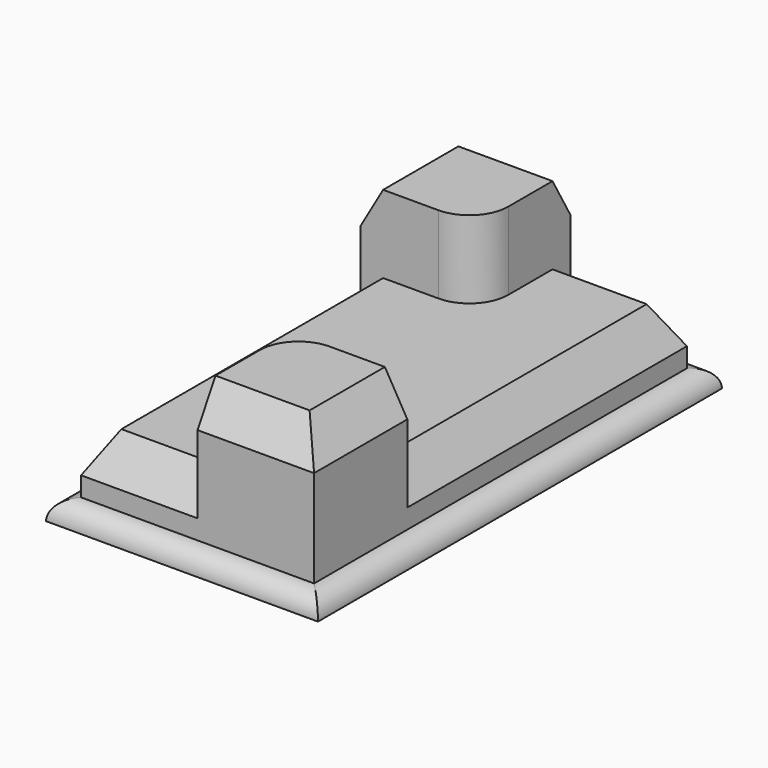
from build123d import *

# Parameters (mm, degrees)
F1_DEPTH = 25.4
F2_DEPTH = 50.8
F0_W     = 88.899994537
F0_H     = 165.099994537
F3_DEPTH = 6.35
F4_R     = 6.34999
F5_SIZE2 = 12.7
F5_SIZE  = 7.3323484187
F6_SIZE2 = 12.7
F6_SIZE  = 7.3323484187
F7_SIZE2 = 12.7
F7_SIZE  = 7.3323484187


# Not quite as in the source:
# - a fillet or chamfer is up to 0.001 mm smaller than in the source, because OpenCascade refuses the exact size


with BuildPart() as f1:
    # F0 (on Top) → F1 (new body)
    with BuildSketch(Plane.XY):
        with BuildLine():
            Line((33.5931509164, 79.879438831), (-4.5068490836, 79.879438831))
            Line((-4.5068490836, 79.879438831), (-4.5068490836, 54.479438831))
            ThreePointArc((-4.5068490836, 54.479438831), (-8.2265929625, 45.49918271), (-17.2068490836, 41.779438831))
            Line((-17.2068490836, 41.779438831), (-42.6068490836, 41.779438831))
            Line((-42.6068490836, 41.779438831), (-42.6068490836, -72.520561169))
            Line((-42.6068490836, -72.520561169), (-4.5068490836, -72.520561169))
            Line((-4.5068490836, -72.520561169), (-4.5068490836, -47.120561169))
            ThreePointArc((-4.5068490836, -47.120561169), (-0.7871052047, -38.1403050479), (8.1931509164, -34.420561169))
            Line((8.1931509164, -34.420561169), (33.5931509164, -34.420561169))
            Line((33.5931509164, -34.420561169), (33.5931509164, 79.879438831))
        make_face()
        with BuildLine():
            Line((33.5931509164, -72.520561169), (33.5931509164, -34.420561169))
            Line((33.5931509164, -34.420561169), (8.1931509164, -34.420561169))
            ThreePointArc((8.1931509164, -34.420561169), (-0.7871052047, -38.1403050479), (-4.5068490836, -47.120561169))
            Line((-4.5068490836, -47.120561169), (-4.5068490836, -72.520561169))
            Line((-4.5068490836, -72.520561169), (33.5931509164, -72.520561169))
        make_face()
        with BuildLine():
            Line((-4.5068490836, 79.879438831), (-42.6068490836, 79.879438831))
            Line((-42.6068490836, 79.879438831), (-42.6068490836, 41.779438831))
            Line((-42.6068490836, 41.779438831), (-17.2068490836, 41.779438831))
            ThreePointArc((-17.2068490836, 41.779438831), (-8.2265929625, 45.49918271), (-4.5068490836, 54.479438831))
            Line((-4.5068490836, 54.479438831), (-4.5068490836, 79.879438831))
        make_face()
    extrude(amount=F1_DEPTH)

    # F0 (on Top) → F2 (join)
    with BuildSketch(Plane.XY):
        with BuildLine():
            Line((33.5931509164, -72.520561169), (33.5931509164, -34.420561169))
            Line((33.5931509164, -34.420561169), (8.1931509164, -34.420561169))
            ThreePointArc((8.1931509164, -34.420561169), (-0.7871052047, -38.1403050479), (-4.5068490836, -47.120561169))
            Line((-4.5068490836, -47.120561169), (-4.5068490836, -72.520561169))
            Line((-4.5068490836, -72.520561169), (33.5931509164, -72.520561169))
        make_face()
        with BuildLine():
            Line((-4.5068490836, 79.879438831), (-42.6068490836, 79.879438831))
            Line((-42.6068490836, 79.879438831), (-42.6068490836, 41.779438831))
            Line((-42.6068490836, 41.779438831), (-17.2068490836, 41.779438831))
            ThreePointArc((-17.2068490836, 41.779438831), (-8.2265929625, 45.49918271), (-4.5068490836, 54.479438831))
            Line((-4.5068490836, 54.479438831), (-4.5068490836, 79.879438831))
        make_face()
    extrude(amount=F2_DEPTH)

    # F0 (on Top) → F3 (join)
    with BuildSketch(Plane.XY):
        with Locations((-4.5068490836, 3.679438831)):
            Rectangle(F0_W, F0_H)
        Polygon((-42.6068490836, 41.779438831), (-42.6068490836, 79.879438831), (-4.5068490836, 79.879438831), (33.5931509164, 79.879438831), (33.5931509164, -34.420561169), (33.5931509164, -72.520561169), (-4.5068490836, -72.520561169), (-42.6068490836, -72.520561169), align=None, mode=Mode.SUBTRACT)
    extrude(amount=F3_DEPTH)

    # F4 (radius 6.35 in the source; OpenCascade refuses exactly that, so slightly less here)
    f4_edges = [f1.edges().sort_by_distance(p)[0] for p in [
        (-4.506849, -78.870558, 6.35),
        (39.943148, 3.679439, 6.35),
        (-48.956846, 3.679439, 6.35),
        (-4.506849, 86.229436, 6.35),
    ]]
    fillet(f4_edges, radius=F4_R)

    # F5
    f5_edges = [f1.edges().sort_by_distance(p)[0] for p in [
        (33.593151, 22.729439, 25.4),
        (14.543151, 79.879439, 25.4),
        (-23.556849, -72.520561, 25.4),
        (-42.606849, -15.370561, 25.4),
    ]]
    f5_side = f1.faces().sort_by_distance((-4.506849, 3.679439, 25.4))[0]
    chamfer(f5_edges, length=F5_SIZE, length2=F5_SIZE2, reference=f5_side)

    # F6
    f6_edges = [f1.edges().sort_by_distance(p)[0] for p in [
        (14.543151, -72.520561, 50.8),
        (33.593151, -53.470561, 50.8),
    ]]
    f6_side = f1.faces().sort_by_distance((14.939193, -53.866603, 50.8))[0]
    chamfer(f6_edges, length=F6_SIZE, length2=F6_SIZE2, reference=f6_side)

    # F7
    f7_edges = [f1.edges().sort_by_distance(p)[0] for p in [
        (-23.556849, 79.879439, 50.8),
        (-42.606849, 60.829439, 50.8),
    ]]
    f7_side = f1.faces().sort_by_distance((-23.952891, 61.225481, 50.8))[0]
    chamfer(f7_edges, length=F7_SIZE, length2=F7_SIZE2, reference=f7_side)


solid = f1.part
